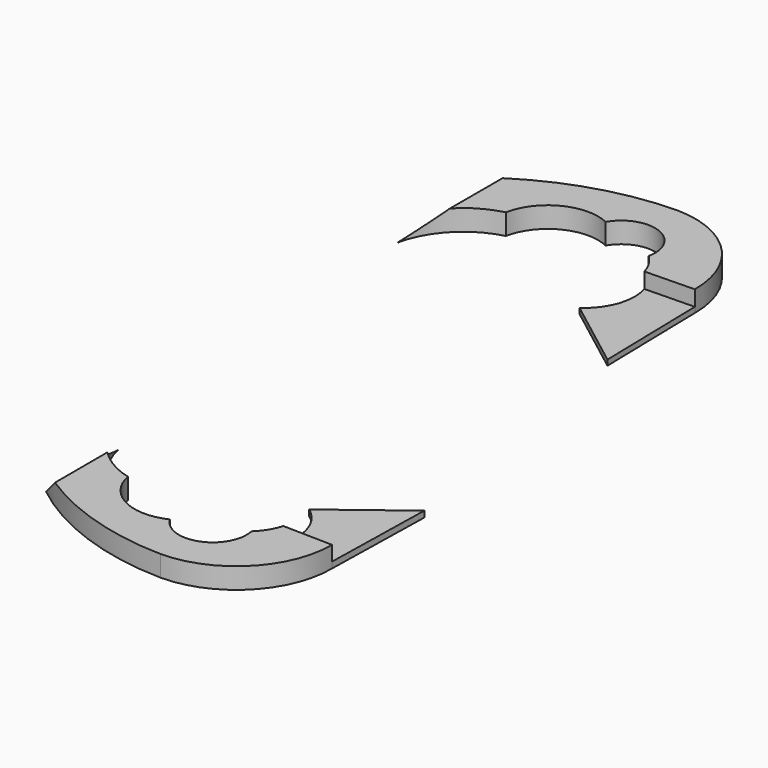
from build123d import *

# Parameters (mm, degrees)
F1_DEPTH    = 7.9375
F3_DEPTH    = 7.9375
F4_T1_DEPTH = 89.6707225602
F5_T1_DEPTH = 89.6707225602
F6_W        = 42.724798455
F6_H        = 5.6216642056
F7_DEPTH    = 27.68579
F8_W        = 42.724798455
F8_H        = 5.8633778039
F9_DEPTH    = 27.94


# Not quite as in the source:
# - a fillet or chamfer that OpenCascade refuses, or shapes differently, is made with other operations: its cross-section is extruded or revolved along the edge and cut away or added
# - a length typed as a fraction of an inch, garbled in the dataset ("3 / 203.2 mm" for 3/8 in), is restored


with BuildPart() as f1:
    # F0 (on Top) → F1 (new body)
    with BuildSketch(Plane.XY):
        with BuildLine():
            ThreePointArc((-49.4316077378, -40.5605532146), (-20.6567184189, -56.5706012946), (11.7271985223, -62.5369920277))
            ThreePointArc((11.7271985223, -62.5369920277), (37.3293245519, -51.810465344), (47.798260752, -26.1019335546))
            Line((47.798260752, -26.1019335546), (48.7327455768, 16.612644064))
            Line((48.7327455768, 16.612644064), (21.5177623814, -4.1354143294))
            ThreePointArc((21.5177623814, -4.1354143294), (29.7231324258, -18.6812958766), (23.6975439262, -34.2570157889))
            ThreePointArc((23.6975439262, -34.2570157889), (15.7671543171, -48.9661744477), (0, -43.4301765663))
            ThreePointArc((0, -43.4301765663), (-16.8413888709, -43.1760896289), (-26.9784570219, -29.7248150211))
            ThreePointArc((-26.9784570219, -29.7248150211), (-41.6350091938, -21.1503252784), (-49.4833397007, -6.0924335212))
            Line((-49.4833397007, -6.0924335212), (-49.4316077378, -40.5605532146))
        make_face()
    extrude(amount=F1_DEPTH)

    # F4: chamfer of 7.9502 on 1 edges, made by hand

    # F4_s2 → F4_t1 (cut)
    with BuildSketch(Plane(origin=(-0.0431333008, 28.7389786103, 0), x_dir=(0, 0, 1), z_dir=(0.0015008624, -0.9999988737, 0))):
        Polygon((-0.0127, 49.4924278722), (7.9375, 41.5422278722), (7.9375, 49.4924278722), align=None)
    extrude(amount=F4_T1_DEPTH, mode=Mode.SUBTRACT)

    # F6 (on face) → F7 (cut)
    with BuildSketch(Plane(origin=(48.3461642406, -1.0576894198, 0), x_dir=(0.021872188, 0.9997607751, 0), z_dir=(0.9997607751, -0.021872188, 0))):
        with Locations((-3.6878375481, 5.1266678972)):
            Rectangle(F6_W, F6_H)
    extrude(amount=-F7_DEPTH, mode=Mode.SUBTRACT)


with BuildPart() as f3:
    # F2 (on Top) → F3 (new body)
    with BuildSketch(Plane.XY):
        with BuildLine():
            ThreePointArc((-45.513824769, 173.2260384447), (-35.376756618, 186.6773130525), (-18.5353677471, 186.9313999898))
            ThreePointArc((-18.5353677471, 186.9313999898), (-2.76821343, 192.4673978713), (5.1621761791, 177.7582392125))
            ThreePointArc((5.1621761791, 177.7582392125), (11.1877646787, 162.1825193002), (2.9823946343, 147.6366377529))
            Line((2.9823946343, 147.6366377529), (30.1973778297, 126.8885793596))
            Line((30.1973778297, 126.8885793596), (29.2628930049, 169.6031569781))
            ThreePointArc((29.2628930049, 169.6031569781), (18.7939568048, 195.3116887676), (-6.8081692248, 206.0382154513))
            ThreePointArc((-6.8081692248, 206.0382154513), (-39.192086166, 200.0718247182), (-67.9669754849, 184.0617766382))
            Line((-67.9669754849, 184.0617766382), (-68.0187074477, 149.5936569448))
            ThreePointArc((-68.0187074477, 149.5936569448), (-60.1703769409, 164.651548702), (-45.513824769, 173.2260384447))
        make_face()
    extrude(amount=F3_DEPTH)

    # F5: chamfer of 7.9502 on 1 edges, made by hand

    # F5_s2 → F5_t1 (cut)
    with BuildSketch(Plane(origin=(0.306783709, 204.4047241236, 0), x_dir=(0, 0, 1), z_dir=(-0.0015008624, -0.9999988737, 0))):
        Polygon((-0.0127, 68.2431503326), (7.9375, 60.2929503326), (7.9375, 68.2431503326), align=None)
    extrude(amount=F5_T1_DEPTH, mode=Mode.SUBTRACT)

    # F8 (on face) → F9 (cut)
    with BuildSketch(Plane(origin=(32.9575985639, 0.7210272801, 0), x_dir=(-0.021872188, 0.9997607751, 0), z_dir=(0.9997607751, 0.021872188, 0))):
        with Locations((147.5601409515, 5.005811098)):
            Rectangle(F8_W, F8_H)
    extrude(amount=-F9_DEPTH, mode=Mode.SUBTRACT)


solid = Compound([f1.part, f3.part])
